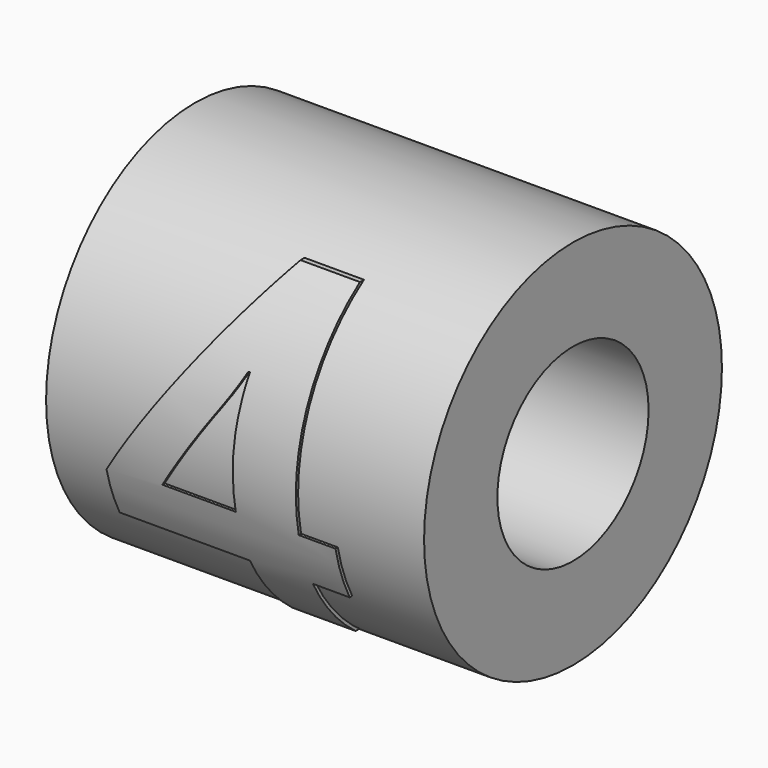
from build123d import *

# Parameters (mm, degrees)
F0_R         = 1
F0_R_2       = 0.985
F0_R_3       = 0.5
F1_DEPTH     = 2
F2_TEXT_SIZE = 2.2604994431
F3_REACH     = 3.0218926603
F4_DEPTH     = 2


# Not quite as in the source:
# - Text() gives the source's letters only with a copy of the font that has no kerning and outlines rounded to 1/6400 em; it was checked with that copy


with BuildPart() as f1:
    # F0 (on Right) → F1 (new body)
    with BuildSketch(Plane.YZ):
        Circle(F0_R)
        Circle(F0_R_2, mode=Mode.SUBTRACT)
        Circle(F0_R_2)
        Circle(F0_R_3, mode=Mode.SUBTRACT)
    extrude(amount=F1_DEPTH)

    f3_end = f1.faces().sort_by_distance((1, -1, 0))[0]
    # F2 (on Front) → F3 (intersect, up to a face of the model that its end follows)
    with BuildSketch(Plane.XZ):
        with Locations((0.2728080435, -0.7963191019)):
            Text('4', F2_TEXT_SIZE, font='Open Sans', font_style=FontStyle.BOLD, text_align=(TextAlign.LEFT, TextAlign.BOTTOM))
    f3_long = extrude(amount=F3_REACH, mode=Mode.PRIVATE)
    add(split(f3_long, bisect_by=f3_end, keep=Keep.BOTTOM, mode=Mode.PRIVATE), mode=Mode.INTERSECT)


with BuildPart() as f4:
    # F0 (on Right) → F4 (new body)
    with BuildSketch(Plane.YZ):
        Circle(F0_R_2)
        Circle(F0_R_3, mode=Mode.SUBTRACT)
    extrude(amount=F4_DEPTH)


solid = Compound([f1.part, f4.part])
